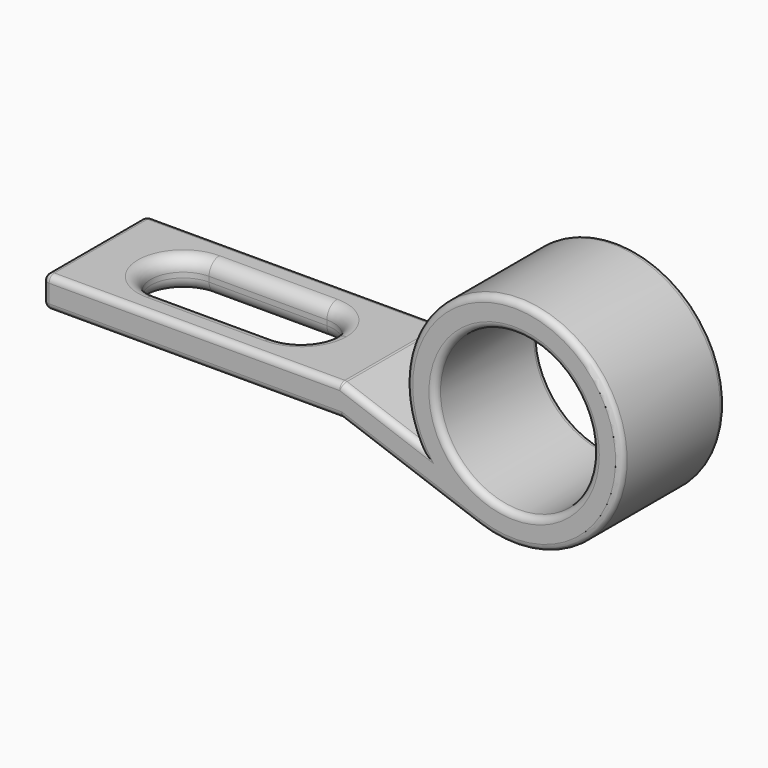
from build123d import *

# Parameters (mm, degrees)
F0_W         = 230.6640344313
F0_H         = 23.9703460229
F0_R         = 60.9213413602
F1_DEPTH     = 100
F2_R         = 5
F3_R         = 5
F5_DEPTH     = 126.802245155
F6_R         = 10
F7_T1_DEPTH  = 90
F7_S5_W      = 5
F7_S5_H      = 5
F7_T6_DEPTH  = 5
F7_S11_W     = 5
F7_S11_H     = 5
F7_T12_DEPTH = 5
F8_R         = 5


# Not quite as in the source:
# - a fillet or chamfer that OpenCascade refuses, or shapes differently, is made with other operations: its cross-section is extruded or revolved along the edge and cut away or added


with BuildPart() as f1:
    # F0 (on Front) → F1 (new body)
    with BuildSketch(Plane.XZ):
        with Locations((18.3448529433, -28.5856171006)):
            Rectangle(F0_W, F0_H)
        with BuildLine():
            Line((193.4351235014, -38.0532068809), (133.676870159, -16.6004440891))
            Line((133.676870159, -16.6004440891), (133.676870159, -40.570790112))
            Line((133.676870159, -40.570790112), (239.5329796232, -78.572335997))
            ThreePointArc((239.5329796232, -78.572335997), (322.8543506597, 62.7027303843), (193.4351235014, -38.0532068809))
        make_face()
        with Locations((267.7398563617, 0)):
            Circle(F0_R, mode=Mode.SUBTRACT)
    extrude(amount=F1_DEPTH)

    # F2
    f2_edges = [f1.edges().sort_by_distance(p)[0] for p in [
        (186.604925, 0, -59.571563),
        (18.344853, 0, -40.57079),
        (18.344853, 0, -16.600444),
        (163.555997, 0, -27.326825),
        (-96.987164, -50, -16.600444),
        (-96.987164, 0, -28.585617),
        (206.818515, -100, 0),
        (322.854351, -100, 62.70273),
        (18.344853, -100, -16.600444),
        (-96.987164, -100, -28.585617),
        (18.344853, -100, -40.57079),
        (186.604925, -100, -59.571563),
        (163.555997, -100, -27.326825),
    ]]
    fillet(f2_edges, radius=F2_R)

    # F3
    f3_edges = [f1.edges().sort_by_distance(p)[0] for p in [
        (206.818515, 0, 0),
    ]]
    fillet(f3_edges, radius=F3_R)

    # F4 (on Top) → F5 (cut)
    with BuildSketch(Plane.XY):
        with BuildLine():
            ThreePointArc((-28.2667462326, -75), (-10.5890767029, -67.6776695297), (-3.2667462326, -50))
            ThreePointArc((-3.2667462326, -50), (-10.5890767029, -32.3223304703), (-28.2667462326, -25))
            ThreePointArc((-28.2667462326, -25), (-53.2667462326, -50), (-28.2667462326, -75))
        make_face()
        with BuildLine():
            ThreePointArc((-28.2667462326, -25), (-10.5890767029, -32.3223304703), (-3.2667462326, -50))
            ThreePointArc((-3.2667462326, -50), (-10.5890767029, -67.6776695297), (-28.2667462326, -75))
            Line((-28.2667462326, -75), (62.8826200036, -75))
            ThreePointArc((62.8826200036, -75), (37.8826200036, -50), (62.8826200036, -25))
            Line((62.8826200036, -25), (-28.2667462326, -25))
        make_face()
        with BuildLine():
            ThreePointArc((87.8826200036, -50), (80.5602895333, -32.3223304703), (62.8826200036, -25))
            ThreePointArc((62.8826200036, -25), (37.8826200036, -50), (62.8826200036, -75))
            ThreePointArc((62.8826200036, -75), (80.5602895333, -67.6776695297), (87.8826200036, -50))
        make_face()
    extrude(amount=-F5_DEPTH, mode=Mode.SUBTRACT)

    # F6
    f6_edges = [f1.edges().sort_by_distance(p)[0] for p in [
        (17.307937, -75, -40.57079),
        (17.307937, -25, -16.600444),
    ]]
    fillet(f6_edges, radius=F6_R)

    # F7: fillet of radius 5 on 1 edges, made by hand

    # F7_s2 → F7_t1 (cut)
    with BuildSketch(Plane.XZ.offset(5)):
        with BuildLine():
            ThreePointArc((-91.9871642723, -40.570790112), (-95.5226981783, -39.106324018), (-96.9871642723, -35.570790112))
            Line((-96.9871642723, -35.570790112), (-96.9871642723, -40.570790112))
            Line((-96.9871642723, -40.570790112), (-91.9871642723, -40.570790112))
        make_face()
    extrude(amount=F7_T1_DEPTH, mode=Mode.SUBTRACT)


with BuildPart() as f7_tool4:
    # F7_s5 → F7_t6 (new body)
    with BuildSketch(Plane.XY.offset(-35.570790112)):
        with Locations((-94.4871642723, -2.5)):
            Rectangle(F7_S5_W, F7_S5_H)
    extrude(amount=-F7_T6_DEPTH)

    # F7_s7 → F7_t8 (revolve, cut)
    with BuildSketch(Plane(origin=(-91.9871642723, -5, -35.570790112), x_dir=(0.7071067812, -0.7071067812, 0), z_dir=(0.7071067812, 0.7071067812, 0))):
        with BuildLine():
            ThreePointArc((0, -5), (5, 0), (0, 5))
            Line((0, 5), (0, -5))
        make_face()
    revolve(axis=Axis((-91.9871642723, -5, -35.570790112), (0, 0, -1)), mode=Mode.SUBTRACT)


with BuildPart() as f1_1:
    add(f1.part)

    # F7_t3: cut F7_tool4
    add(f7_tool4.part, mode=Mode.SUBTRACT)


with BuildPart() as f7_tool10:
    # F7_s11 → F7_t12 (new body)
    with BuildSketch(Plane.XY.offset(-35.570790112)):
        with Locations((-94.4871642723, -97.5)):
            Rectangle(F7_S11_W, F7_S11_H)
    extrude(amount=-F7_T12_DEPTH)

    # F7_s13 → F7_t14 (revolve, cut)
    with BuildSketch(Plane(origin=(-91.9871642723, -95, -35.570790112), x_dir=(0.7071067812, 0.7071067812, 0), z_dir=(-0.7071067812, 0.7071067812, 0))):
        with BuildLine():
            ThreePointArc((0, -5), (5, 0), (0, 5))
            Line((0, 5), (0, -5))
        make_face()
    revolve(axis=Axis((-91.9871642723, -95, -35.570790112), (0, 0, -1)), mode=Mode.SUBTRACT)


with BuildPart() as f1_2:
    add(f1_1.part)

    # F7_t9: cut F7_tool10
    add(f7_tool10.part, mode=Mode.SUBTRACT)

    # F8
    f8_edges = [f1_2.edges().sort_by_distance(p)[0] for p in [
        (133.67687, -50, -40.57079),
        (133.67687, -50, -16.600444),
    ]]
    fillet(f8_edges, radius=F8_R)


solid = f1_2.part
